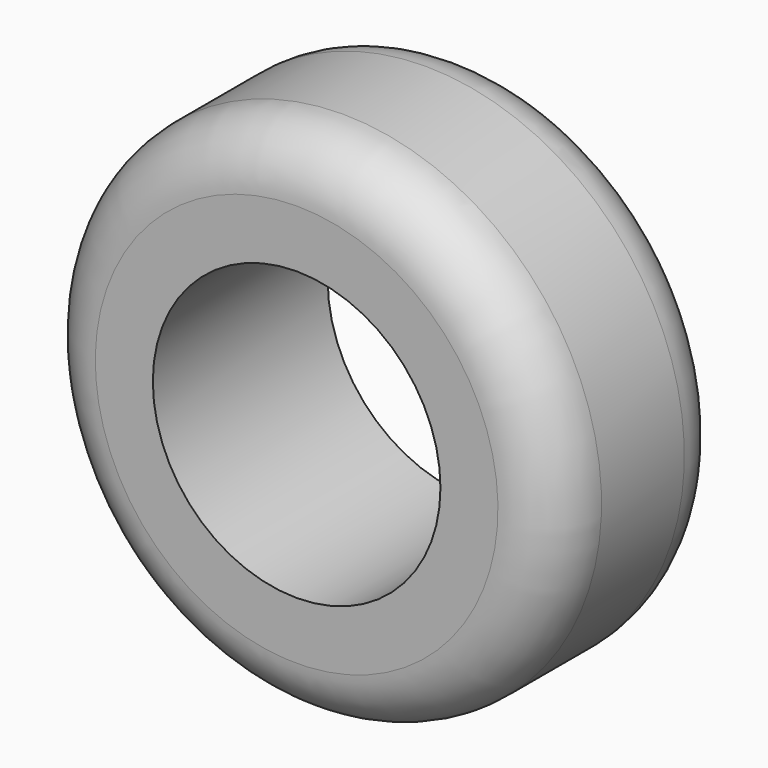
from build123d import *


# Not quite as in the source:
# - a feature names something its author has since deleted; it is built from what else it names


with BuildPart() as f2:
    # F0 (on Right) → F2 (revolve)
    with BuildSketch(Plane.YZ):
        with BuildLine():
            ThreePointArc((-0.95, 1.45), (-1.6571067812, 1.1571067812), (-1.95, 0.45))
            Line((-1.95, 0.45), (-1.95, -0.55))
            Line((-1.95, -0.55), (1.85, -0.55))
            Line((1.85, -0.55), (1.85, 0.45))
            ThreePointArc((1.85, 0.45), (1.5571067812, 1.1571067812), (0.85, 1.45))
            Line((0.85, 1.45), (-0.95, 1.45))
        make_face()
    revolve(axis=Axis((0, 0.1895423047, -3.05), (0, 1, 0)))


solid = f2.part
